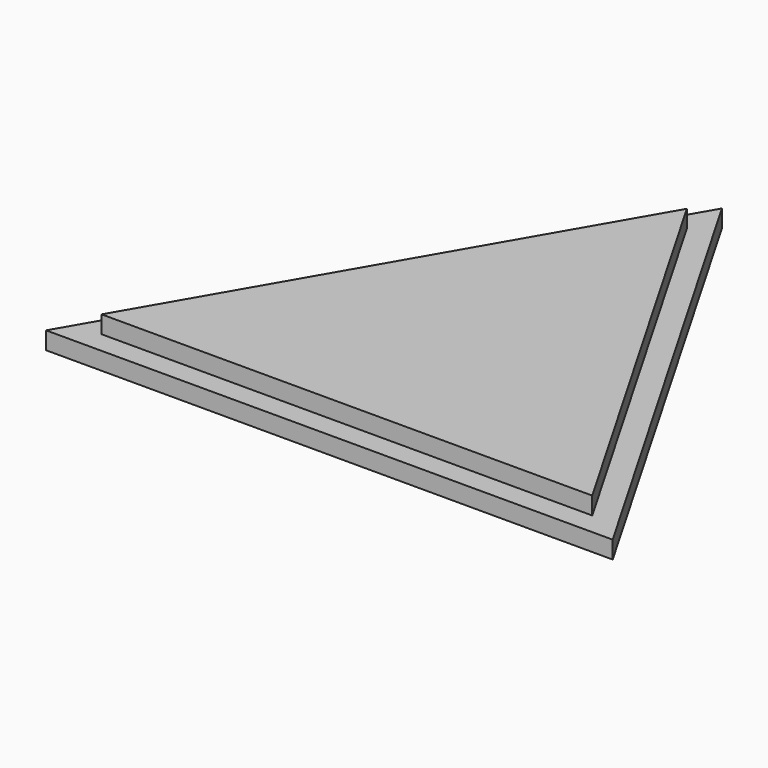
from build123d import *

# Parameters (mm, degrees)
F1_DEPTH = 4
F2_DEPTH = 2
F3_START = 2
F3_DEPTH = 2
F4_SIZE  = 1.99999


# Not quite as in the source:
# - a fillet or chamfer is up to 0.001 mm smaller than in the source, because OpenCascade refuses the exact size


with BuildPart() as f1:
    # F0 (on Top) → F1 (new body)
    with BuildSketch(Plane.XY):
        Polygon((32.7846783229, 14.824549064), (4.8026783229, 63.2907947614), (-23.1793216771, 14.824549064), align=None)
        Polygon((-19.715220062, 16.824549064), (4.8026783229, 59.2907947614), (29.3205767077, 16.824549064), align=None, mode=Mode.SUBTRACT)
    extrude(amount=F1_DEPTH)

    # F0 (on Top) → F2 (join)
    with BuildSketch(Plane.XY):
        Polygon((37.1148053418, 12.324549064), (4.8026783229, 68.2907947614), (-27.509448696, 12.324549064), align=None)
        Polygon((-23.1793216771, 14.824549064), (4.8026783229, 63.2907947614), (32.7846783229, 14.824549064), align=None, mode=Mode.SUBTRACT)
    extrude(amount=F2_DEPTH)

    # F0 (on Top) → F3 (join)
    with BuildSketch(Plane.XY.offset(F3_START)):
        Polygon((29.3205767077, 16.824549064), (4.8026783229, 59.2907947614), (-19.715220062, 16.824549064), align=None)
    extrude(amount=F3_DEPTH)

    # F4 (size 2 in the source; OpenCascade refuses exactly that, so slightly less here)
    f4_edges = [f1.edges().sort_by_distance(p)[0] for p in [
        (4.802678, 16.824549, 0),
        (-7.456271, 38.057672, 0),
        (17.061628, 38.057672, 0),
    ]]
    chamfer(f4_edges, length=F4_SIZE)


solid = f1.part
